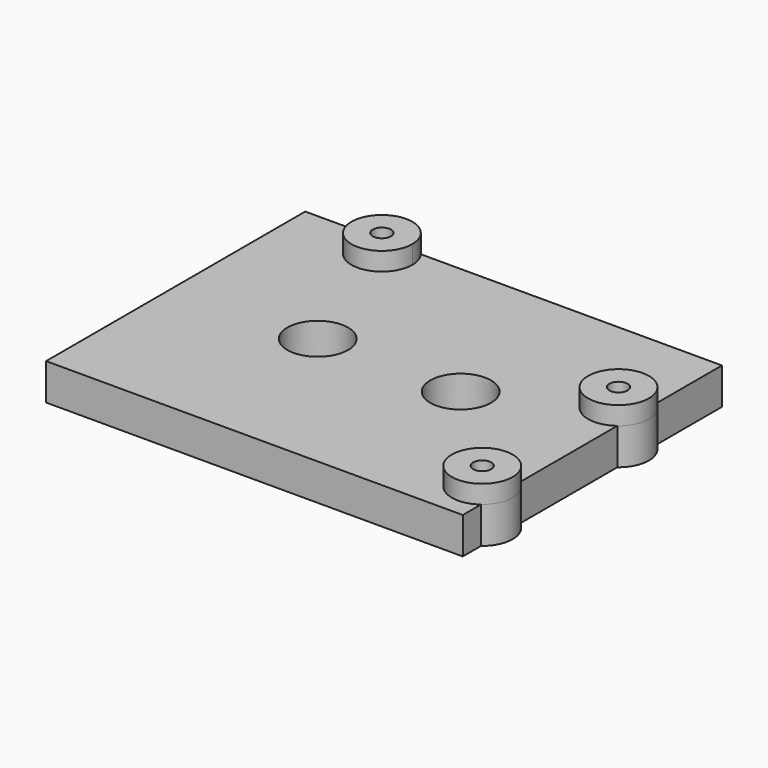
from build123d import *
from build123d import SkipClean  # not in build123d's __all__

# Parameters (mm, degrees)
F0_R     = 5
F0_R_2   = 1.5
F1_DEPTH = 6
F2_R     = 1.5
F3_DEPTH = 3


# Not quite as in the source:
# - a feature names something its author has since deleted; it is built from what else it names


with BuildPart() as f1:
    # F0 (on Top) → F1 (new body)
    with BuildSketch(Plane.XY):
        with BuildLine():
            Line((42.65, 26.625), (11.4, 26.625))
            Line((11.4, 26.625), (-3.85, 26.625))
            ThreePointArc((-3.85, 26.625), (-7.85, 28.625), (-11.85, 26.625))
            Line((-11.85, 26.625), (-22.85, 26.625))
            Line((-22.85, 26.625), (-22.85, -26.625))
            Line((-22.85, -26.625), (45.65, -26.625))
            Line((45.65, -26.625), (45.65, -22.875))
            ThreePointArc((45.65, -22.875), (47.65, -18.875), (45.65, -14.875))
            Line((45.65, -14.875), (45.65, 5.125))
            ThreePointArc((45.65, 5.125), (47.65, 9.125), (45.65, 13.125))
            Line((45.65, 13.125), (45.65, 26.625))
            Line((45.65, 26.625), (42.65, 26.625))
        make_face()
        with Locations((0.5, 0)):
            Circle(F0_R, mode=Mode.SUBTRACT)
        with Locations((42.65, -18.875)):
            Circle(F0_R_2, mode=Mode.SUBTRACT)
        with BuildLine():
            ThreePointArc((29, 0), (24, -5), (19, 0))
            ThreePointArc((19, 0), (24, 5), (29, 0))
        make_face(mode=Mode.SUBTRACT)
        with BuildLine():
            ThreePointArc((-7.85, 25.125), (-6.7893398282, 24.6856601718), (-6.35, 23.625))
            ThreePointArc((-6.35, 23.625), (-8.9106601718, 22.5643398282), (-7.85, 25.125))
        make_face(mode=Mode.SUBTRACT)
        with Locations((42.65, 9.125)):
            Circle(F0_R_2, mode=Mode.SUBTRACT)
    extrude(amount=F1_DEPTH)

    # F2 (on face) → F3 (join)
    with BuildSketch(Plane.XY.offset(6)):
        with BuildLine():
            ThreePointArc((-11.85, 26.625), (-9.4311388301, 18.8815835097), (-2.85, 23.625))
            ThreePointArc((-2.85, 23.625), (-3.1065835097, 25.2061388301), (-3.85, 26.625))
            ThreePointArc((-3.85, 26.625), (-7.85, 28.625), (-11.85, 26.625))
        make_face()
        with Locations((-7.85, 23.625)):
            Circle(F2_R, mode=Mode.SUBTRACT)
        with BuildLine():
            ThreePointArc((47.65, 9.125), (47.122135955, 11.3610679775), (45.65, 13.125))
            ThreePointArc((45.65, 13.125), (37.65, 9.125), (45.65, 5.125))
            ThreePointArc((45.65, 5.125), (47.122135955, 6.8889320225), (47.65, 9.125))
        make_face()
        with Locations((42.65, 9.125)):
            Circle(F2_R, mode=Mode.SUBTRACT)
        with BuildLine():
            ThreePointArc((47.65, -18.875), (47.122135955, -16.6389320225), (45.65, -14.875))
            ThreePointArc((45.65, -14.875), (37.65, -18.875), (45.65, -22.875))
            ThreePointArc((45.65, -22.875), (47.122135955, -21.1110679775), (47.65, -18.875))
        make_face()
        with Locations((42.65, -18.875)):
            Circle(F2_R, mode=Mode.SUBTRACT)
    with SkipClean():  # cleaning this boolean's faces spoils the solid; the shape is the same uncleaned
        extrude(amount=F3_DEPTH)


solid = f1.part
